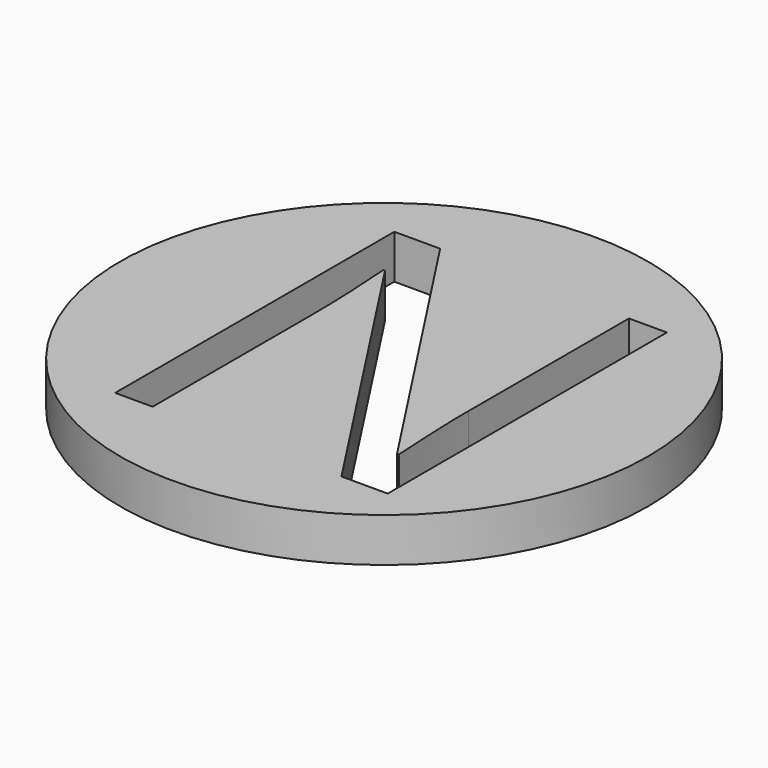
from build123d import *

# Parameters (mm, degrees)
F0_R         = 12
F1_DEPTH     = 2
F2_TEXT_SIZE = 22.2222222222
F3_DEPTH     = 25


# Not quite as in the source:
# - Text() gives the source's letters only with a copy of the font that has no kerning and outlines rounded to 1/6400 em; it was checked with that copy


with BuildPart() as f1:
    # F0 (on Top) → F1 (new body)
    with BuildSketch(Plane.XY):
        Circle(F0_R)
    extrude(amount=F1_DEPTH)

    # F2 (on face) → F3 (cut)
    with BuildSketch(Plane.XY.offset(2)):
        with Locations((-8.0069444444, -8)):
            Text('N', F2_TEXT_SIZE, font='Open Sans', text_align=(TextAlign.LEFT, TextAlign.BOTTOM))
    extrude(amount=-F3_DEPTH, mode=Mode.SUBTRACT)


solid = f1.part
